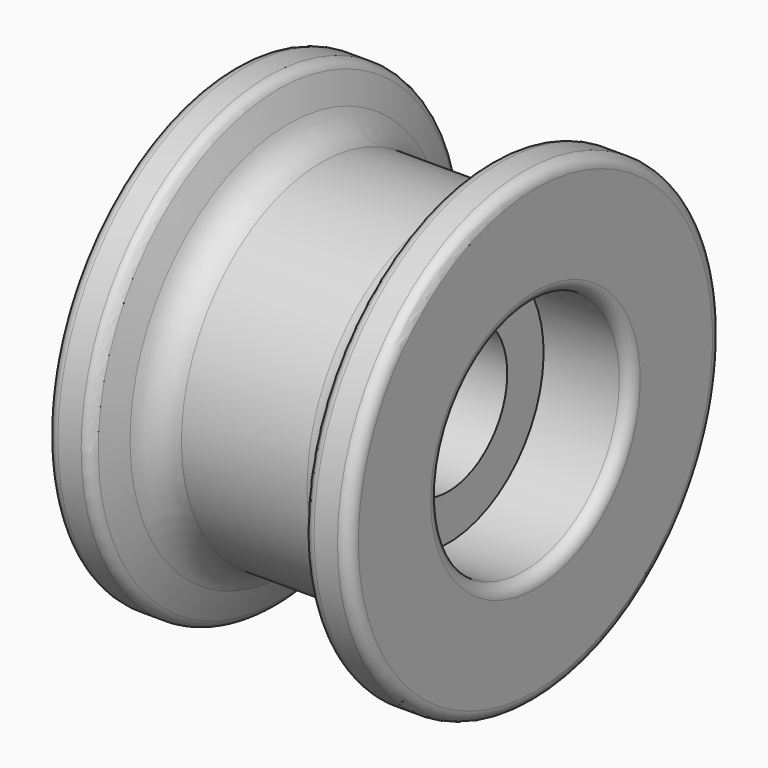
from build123d import *

# Parameters (mm, degrees)
F0_W = 0.6
F0_H = 3.175


# Not quite as in the source:
# - a feature names something its author has since deleted; it is built from what else it names


with BuildPart() as f1:
    # F0 (on Front) → F1 (revolve)
    with BuildSketch(Plane.XZ):
        with BuildLine():
            Line((-5, 10), (-6, 10))
            ThreePointArc((-6, 10), (-6.3535533906, 9.8535533906), (-6.5, 9.5))
            Line((-6.5, 9.5), (-6.5, 5.625))
            ThreePointArc((-6.5, 5.625), (-6.3535533906, 5.2714466094), (-6, 5.125))
            Line((-6, 5.125), (-2.75, 5.125))
            Line((-2.75, 5.125), (-2.75, 3.175))
            Line((-2.75, 3.175), (-2.15, 3.175))
            Line((-2.15, 3.175), (0, 3.175))
            Line((0, 3.175), (2.75, 3.175))
            Line((2.75, 3.175), (2.75, 5.125))
            Line((2.75, 5.125), (6, 5.125))
            ThreePointArc((6, 5.125), (6.3535533906, 5.2714466094), (6.5, 5.625))
            Line((6.5, 5.625), (6.5, 9.5))
            ThreePointArc((6.5, 9.5), (6.3535533906, 9.8535533906), (6, 10))
            Line((6, 10), (5, 10))
            ThreePointArc((5, 10), (4.7123753868, 9.9089890975), (4.5294586761, 9.6690883275))
            Line((4.5294586761, 9.6690883275), (4.1067378574, 8.4927350176))
            ThreePointArc((4.1067378574, 8.4927350176), (3.5579877254, 7.7730327075), (2.6951138857, 7.5))
            Line((2.6951138857, 7.5), (0, 7.5))
            Line((0, 7.5), (-2.6951138857, 7.5))
            ThreePointArc((-2.6951138857, 7.5), (-3.5579877254, 7.7730327075), (-4.1067378574, 8.4927350176))
            Line((-4.1067378574, 8.4927350176), (-4.5294586761, 9.6690883275))
            ThreePointArc((-4.5294586761, 9.6690883275), (-4.7123753868, 9.9089890975), (-5, 10))
        make_face()
        with Locations((-2.45, 1.5875)):
            Rectangle(F0_W, F0_H)
    revolve(axis=Axis((0.9040212664, 0, 0), (1, 0, 0)))


solid = f1.part
